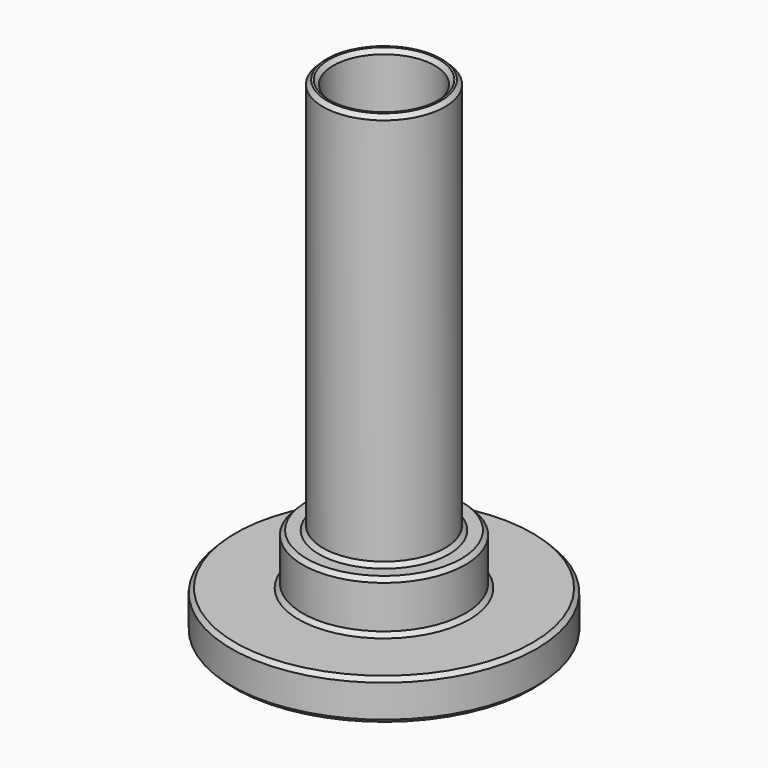
from build123d import *

# Parameters (mm, degrees)
F0_R     = 7.5
F1_DEPTH = 2
F2_R     = 3
F3_DEPTH = 22
F5_D     = 5
F6_R     = 4
F6_R_2   = 3
F7_DEPTH = 2.5
F8_SIZE  = 0.2


with BuildPart() as f1:
    # F0 (on Top) → F1 (new body)
    with BuildSketch(Plane.XY):
        Circle(F0_R)
    extrude(amount=F1_DEPTH)

    # F2 (on face) → F3 (join)
    with BuildSketch(Plane.XY.offset(2)):
        Circle(F2_R)
    extrude(amount=F3_DEPTH)

    # F5 (through all)
    with Locations(Plane(origin=(0, 0, 0), x_dir=(1, 0, 0), z_dir=(0, 0, -1))):
        with Locations((0, 0)):
            Hole(F5_D / 2)

    # F6 (on face) → F7 (join)
    with BuildSketch(Plane.XY.offset(2)):
        Circle(F6_R)
        Circle(F6_R_2, mode=Mode.SUBTRACT)
    extrude(amount=F7_DEPTH)

    # F8
    f8_edges = [f1.edges().sort_by_distance(p)[0] for p in [
        (-3, 0, 24),
        (-7.5, 0, 2),
        (-7.5, 0, 0),
        (-3, 0, 4.5),
        (-4, 0, 4.5),
        (-4, 0, 2),
        (-2.5, 0, 0),
        (-2.5, 0, 24),
    ]]
    chamfer(f8_edges, length=F8_SIZE)


solid = f1.part
